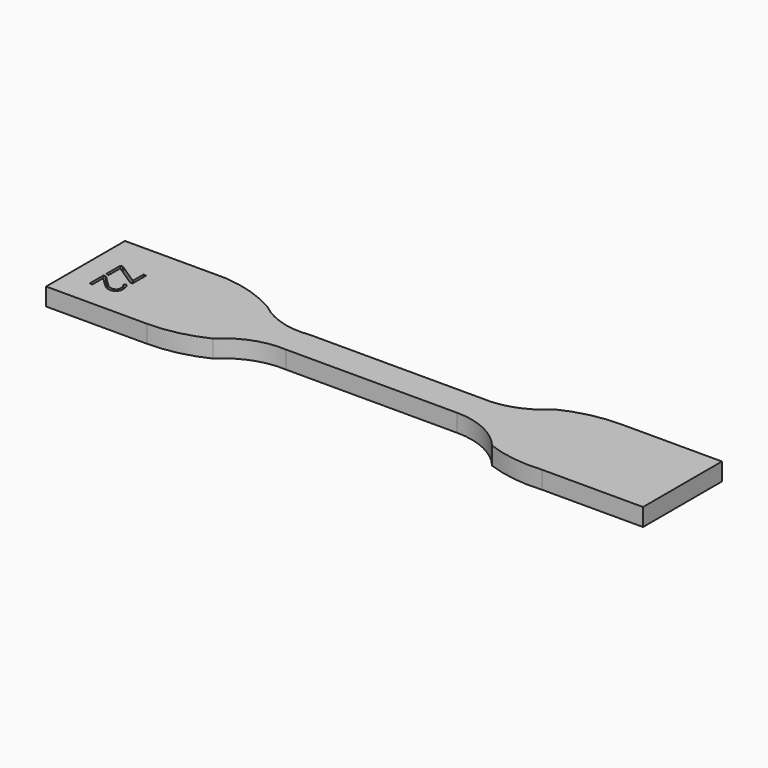
from build123d import *

# Parameters (mm, degrees)
F1_DEPTH     = 3.4
F2_TEXT_SIZE = 7.0564552314
F3_DEPTH     = 1


# Not quite as in the source:
# - Text() gives the source's letters only with a copy of the font that has no kerning and outlines rounded to 1/6400 em; it was checked with that copy


with BuildPart() as f1:
    # F0 (on Top) → F1 (new body)
    with BuildSketch(Plane.XY):
        with BuildLine():
            Line((-14.4320548165, 19.7811394548), (-33.8720548165, 19.7811394548))
            Line((-33.8720548165, 19.7811394548), (-33.8720548165, 0.7811394548))
            Line((-33.8720548165, 0.7811394548), (-14.4320548165, 0.7811394548))
            ThreePointArc((-14.4320548165, 0.7811394548), (-8.9053122052, 1.3996892086), (-3.6520548165, 3.2247301661))
            ThreePointArc((-3.6520548165, 3.2247301661), (1.3014698263, 6.4128780055), (7.1279451835, 7.2811394548))
            Line((7.1279451835, 7.2811394548), (40.1279451835, 7.2811394548))
            ThreePointArc((40.1279451835, 7.2811394548), (46.0837574042, 5.9511158081), (50.9079451835, 2.2137538538))
            ThreePointArc((50.9079451835, 2.2137538538), (56.2191047011, 0.9041953221), (61.6879451835, 0.7811394548))
            Line((61.6879451835, 0.7811394548), (81.1279451835, 0.7811394548))
            Line((81.1279451835, 0.7811394548), (81.1279451835, 19.7811394548))
            Line((81.1279451835, 19.7811394548), (61.6879451835, 19.7811394548))
            ThreePointArc((61.6879451835, 19.7811394548), (56.1612025723, 19.162589701), (50.9079451835, 17.3375487435))
            ThreePointArc((50.9079451835, 17.3375487435), (45.9544205407, 14.1494009041), (40.1279451835, 13.2811394548))
            Line((40.1279451835, 13.2811394548), (7.1279451835, 13.2811394548))
            ThreePointArc((7.1279451835, 13.2811394548), (1.4167452884, 13.6925537245), (-3.6520548165, 16.3560723447))
            ThreePointArc((-3.6520548165, 16.3560723447), (-8.8458057958, 18.686276846), (-14.4320548165, 19.7811394548))
        make_face()
    extrude(amount=F1_DEPTH)

    # F2 (on face) → F3 (cut)
    with BuildSketch(Plane.XY.offset(3.4)):
        with Locations(Location((-29.3720550835, 13.353464842), (0, 0, -90))):
            Text('Z2', F2_TEXT_SIZE, font='Open Sans', text_align=(TextAlign.LEFT, TextAlign.BOTTOM))
    extrude(amount=-F3_DEPTH, mode=Mode.SUBTRACT)


solid = f1.part
